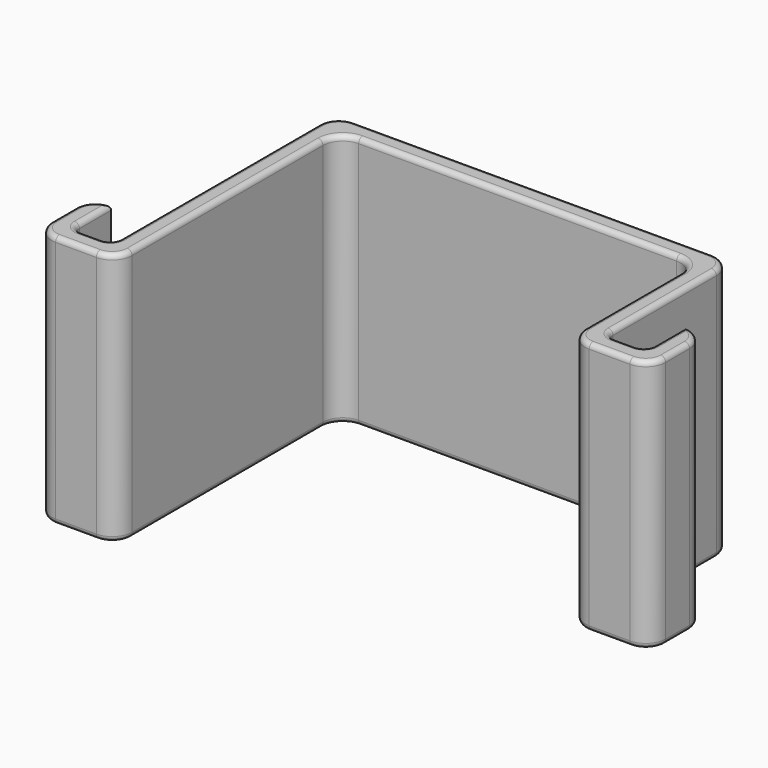
from build123d import *

# Parameters (mm, degrees)
F0_W         = 36
F0_H         = 2
F0_W_2       = 2
F0_W_3       = 4.1
F1_DEPTH     = 25.5
F2_R         = 1.99999
F3_R         = 1
F4_T1_DEPTH  = 36.00002
F4_T3_DEPTH  = 32.00002
F4_T5_DEPTH  = 25.00001
F4_T7_DEPTH  = 2.1
F4_T9_DEPTH  = 5.25
F4_T11_DEPTH = 13.00001
F4_T13_DEPTH = 1.25001
F4_T15_DEPTH = 2.1
F4_T17_DEPTH = 3.00002
F4_T19_DEPTH = 5.25
F4_T21_DEPTH = 4.10002
F4_T23_DEPTH = 1.25001
F4_T25_DEPTH = 24.00002
F4_T27_DEPTH = 3.00002
F4_T29_DEPTH = 4.10002
F4_T31_DEPTH = 12.00002
F4_T34_ANGLE = 90
F4_T36_ANGLE = 90
F4_T38_ANGLE = 90
F4_T40_ANGLE = 90
F4_T42_ANGLE = 90
F4_T44_ANGLE = 90
F4_T46_ANGLE = 90
F4_T48_ANGLE = 90
F4_T50_ANGLE = 90
F4_T52_ANGLE = 90
F4_T54_ANGLE = 90
F4_T56_ANGLE = 90
F4_T58_ANGLE = 90
F4_T60_ANGLE = 90
F4_T62_ANGLE = 90
F4_T64_ANGLE = 90
F4_T66_ANGLE = 90
F4_T68_ANGLE = 90
F4_T70_ANGLE = 90
F4_T72_ANGLE = 90
F4_T74_ANGLE = 90
F4_T76_ANGLE = 90
F4_T78_ANGLE = 90
F4_T80_ANGLE = 90
F4_T82_ANGLE = 90
F4_T84_ANGLE = 90
F4_T86_ANGLE = 90
F4_T88_ANGLE = 90


# Not quite as in the source:
# - a fillet or chamfer that OpenCascade refuses, or shapes differently, is made with other operations: its cross-section is extruded or revolved along the edge and cut away or added
# - a fillet or chamfer is up to 0.001 mm smaller than in the source, because OpenCascade refuses the exact size


with BuildPart() as f1:
    # F0 (on Top) → F1 (new body)
    with BuildSketch(Plane.XY):
        Polygon((0, -2), (0, 0), (-2, 0), (-2, -28), (0, -28), align=None)
        with Locations((18, -1)):
            Rectangle(F0_W, F0_H)
        Polygon((38, 0), (36, 0), (36, -2), (36, -16), (38, -16), align=None)
        with Locations((37, -17)):
            Rectangle(F0_W_2, F0_H)
        with Locations((40.05, -17)):
            Rectangle(F0_W_3, F0_H)
        Polygon((42.1, -11), (42.1, -16), (42.1, -18), (44.1, -18), (44.1, -11), align=None)
        Polygon((0, -30), (0, -28), (-2, -28), (-6.1, -28), (-6.1, -30), align=None)
        Polygon((-6.1, -30), (-6.1, -28), (-6.1, -23), (-8.1, -23), (-8.1, -30), align=None)
    extrude(amount=F1_DEPTH)

    # F2 (radius 2 in the source; OpenCascade refuses exactly that, so slightly less here)
    f2_edges = [f1.edges().sort_by_distance(p)[0] for p in [
        (0, -30, 12.75),
        (36, -18, 12.75),
        (-8.1, -30, 12.75),
        (44.1, -18, 12.75),
        (0, -2, 12.75),
        (36, -2, 12.75),
        (-2, 0, 12.75),
        (38, 0, 12.75),
        (44.1, -11, 12.75),
        (-8.1, -23, 12.75),
    ]]
    fillet(f2_edges, radius=F2_R)

    # F3
    f3_edges = [f1.edges().sort_by_distance(p)[0] for p in [
        (-2, -28, 12.75),
        (-6.1, -28, 12.75),
        (42.1, -16, 12.75),
        (38, -16, 12.75),
    ]]
    fillet(f3_edges, radius=F3_R)

    # F4: fillet of radius 0.5 on 58 edges, made by hand

    # F4_s2 → F4_t1 (cut)
    with BuildSketch(Plane.YZ.offset(-1e-05)):
        with BuildLine():
            ThreePointArc((-0.5, 25.5), (-0.1464466094, 25.3535533906), (0, 25))
            Line((0, 25), (0, 25.5))
            Line((0, 25.5), (-0.5, 25.5))
        make_face()
        with BuildLine():
            ThreePointArc((-0.5, 0), (-0.1464466094, 0.1464466094), (0, 0.5))
            Line((0, 0.5), (0, 0))
            Line((0, 0), (-0.5, 0))
        make_face()
    extrude(amount=F4_T1_DEPTH, mode=Mode.SUBTRACT)

    # F4_s4 → F4_t3 (cut)
    with BuildSketch(Plane.YZ.offset(1.99999)):
        with BuildLine():
            ThreePointArc((-1.5, 0), (-1.8535533906, 0.1464466094), (-2, 0.5))
            Line((-2, 0.5), (-2, 0))
            Line((-2, 0), (-1.5, 0))
        make_face()
        with BuildLine():
            ThreePointArc((-1.5, 25.5), (-1.8535533906, 25.3535533906), (-2, 25))
            Line((-2, 25), (-2, 25.5))
            Line((-2, 25.5), (-1.5, 25.5))
        make_face()
    extrude(amount=F4_T3_DEPTH, mode=Mode.SUBTRACT)

    # F4_s6 → F4_t5 (cut)
    with BuildSketch(Plane.XZ.offset(1.99999)):
        with BuildLine():
            ThreePointArc((-2, 25), (-1.8535533906, 25.3535533906), (-1.5, 25.5))
            Line((-1.5, 25.5), (-2, 25.5))
            Line((-2, 25.5), (-2, 25))
        make_face()
        with BuildLine():
            ThreePointArc((-2, 0.5), (-1.8535533906, 0.1464466094), (-1.5, 0))
            Line((-1.5, 0), (-2, 0))
            Line((-2, 0), (-2, 0.5))
        make_face()
    extrude(amount=F4_T5_DEPTH, mode=Mode.SUBTRACT)

    # F4_s8 → F4_t7 (cut)
    with BuildSketch(Plane.YZ.offset(-5.1)):
        with BuildLine():
            ThreePointArc((-28.5, 25.5), (-28.1464466094, 25.3535533906), (-28, 25))
            Line((-28, 25), (-28, 25.5))
            Line((-28, 25.5), (-28.5, 25.5))
        make_face()
        with BuildLine():
            ThreePointArc((-28.5, 0), (-28.1464466094, 0.1464466094), (-28, 0.5))
            Line((-28, 0.5), (-28, 0))
            Line((-28, 0), (-28.5, 0))
        make_face()
    extrude(amount=F4_T7_DEPTH, mode=Mode.SUBTRACT)

    # F4_s10 → F4_t9 (cut)
    with BuildSketch(Plane.XZ.offset(21.75)):
        with BuildLine():
            ThreePointArc((-6.6, 25.5), (-6.2464466094, 25.3535533906), (-6.1, 25))
            Line((-6.1, 25), (-6.1, 25.5))
            Line((-6.1, 25.5), (-6.6, 25.5))
        make_face()
        with BuildLine():
            ThreePointArc((-6.6, 0), (-6.2464466094, 0.1464466094), (-6.1, 0.5))
            Line((-6.1, 0.5), (-6.1, 0))
            Line((-6.1, 0), (-6.6, 0))
        make_face()
    extrude(amount=F4_T9_DEPTH, mode=Mode.SUBTRACT)

    # F4_s12 → F4_t11 (cut)
    with BuildSketch(Plane.XZ.offset(1.99999)):
        with BuildLine():
            ThreePointArc((37.5, 25.5), (37.8535533906, 25.3535533906), (38, 25))
            Line((38, 25), (38, 25.5))
            Line((38, 25.5), (37.5, 25.5))
        make_face()
        with BuildLine():
            ThreePointArc((37.5, 0), (37.8535533906, 0.1464466094), (38, 0.5))
            Line((38, 0.5), (38, 0))
            Line((38, 0), (37.5, 0))
        make_face()
    extrude(amount=F4_T11_DEPTH, mode=Mode.SUBTRACT)

    # F4_s14 → F4_t13 (cut)
    with BuildSketch(Plane.YZ.offset(-6.10001)):
        with BuildLine():
            ThreePointArc((-23.5, 25.5), (-23.1464466094, 25.3535533906), (-23, 25))
            Line((-23, 25), (-23, 25.5))
            Line((-23, 25.5), (-23.5, 25.5))
        make_face()
        with BuildLine():
            ThreePointArc((-23.5, 0), (-23.1464466094, 0.1464466094), (-23, 0.5))
            Line((-23, 0.5), (-23, 0))
            Line((-23, 0), (-23.5, 0))
        make_face()
    extrude(amount=F4_T13_DEPTH, mode=Mode.SUBTRACT)

    # F4_s16 → F4_t15 (cut)
    with BuildSketch(Plane.YZ.offset(39)):
        with BuildLine():
            ThreePointArc((-16.5, 25.5), (-16.1464466094, 25.3535533906), (-16, 25))
            Line((-16, 25), (-16, 25.5))
            Line((-16, 25.5), (-16.5, 25.5))
        make_face()
        with BuildLine():
            ThreePointArc((-16.5, 0), (-16.1464466094, 0.1464466094), (-16, 0.5))
            Line((-16, 0.5), (-16, 0))
            Line((-16, 0), (-16.5, 0))
        make_face()
    extrude(amount=F4_T15_DEPTH, mode=Mode.SUBTRACT)

    # F4_s18 → F4_t17 (cut)
    with BuildSketch(Plane.XZ.offset(24.99999)):
        with BuildLine():
            ThreePointArc((-7.6, 25.5), (-7.9535533906, 25.3535533906), (-8.1, 25))
            Line((-8.1, 25), (-8.1, 25.5))
            Line((-8.1, 25.5), (-7.6, 25.5))
        make_face()
        with BuildLine():
            ThreePointArc((-7.6, 0), (-7.9535533906, 0.1464466094), (-8.1, 0.5))
            Line((-8.1, 0.5), (-8.1, 0))
            Line((-8.1, 0), (-7.6, 0))
        make_face()
    extrude(amount=F4_T17_DEPTH, mode=Mode.SUBTRACT)

    # F4_s20 → F4_t19 (cut)
    with BuildSketch(Plane.XZ.offset(9.75)):
        with BuildLine():
            ThreePointArc((42.6, 25.5), (42.2464466094, 25.3535533906), (42.1, 25))
            Line((42.1, 25), (42.1, 25.5))
            Line((42.1, 25.5), (42.6, 25.5))
        make_face()
        with BuildLine():
            ThreePointArc((42.6, 0), (42.2464466094, 0.1464466094), (42.1, 0.5))
            Line((42.1, 0.5), (42.1, 0))
            Line((42.1, 0), (42.6, 0))
        make_face()
    extrude(amount=F4_T19_DEPTH, mode=Mode.SUBTRACT)

    # F4_s22 → F4_t21 (cut)
    with BuildSketch(Plane.YZ.offset(-6.10001)):
        with BuildLine():
            ThreePointArc((-29.5, 25.5), (-29.8535533906, 25.3535533906), (-30, 25))
            Line((-30, 25), (-30, 25.5))
            Line((-30, 25.5), (-29.5, 25.5))
        make_face()
        with BuildLine():
            ThreePointArc((-29.5, 0), (-29.8535533906, 0.1464466094), (-30, 0.5))
            Line((-30, 0.5), (-30, 0))
            Line((-30, 0), (-29.5, 0))
        make_face()
    extrude(amount=F4_T21_DEPTH, mode=Mode.SUBTRACT)

    # F4_s24 → F4_t23 (cut)
    with BuildSketch(Plane.YZ.offset(40.85)):
        with BuildLine():
            ThreePointArc((-11.5, 25.5), (-11.1464466094, 25.3535533906), (-11, 25))
            Line((-11, 25), (-11, 25.5))
            Line((-11, 25.5), (-11.5, 25.5))
        make_face()
        with BuildLine():
            ThreePointArc((-11.5, 0), (-11.1464466094, 0.1464466094), (-11, 0.5))
            Line((-11, 0.5), (-11, 0))
            Line((-11, 0), (-11.5, 0))
        make_face()
    extrude(amount=F4_T23_DEPTH, mode=Mode.SUBTRACT)

    # F4_s26 → F4_t25 (cut)
    with BuildSketch(Plane.XZ.offset(3.99999)):
        with BuildLine():
            ThreePointArc((-0.5, 25.5), (-0.1464466094, 25.3535533906), (0, 25))
            Line((0, 25), (0, 25.5))
            Line((0, 25.5), (-0.5, 25.5))
        make_face()
        with BuildLine():
            ThreePointArc((-0.5, 0), (-0.1464466094, 0.1464466094), (0, 0.5))
            Line((0, 0.5), (0, 0))
            Line((0, 0), (-0.5, 0))
        make_face()
    extrude(amount=F4_T25_DEPTH, mode=Mode.SUBTRACT)

    # F4_s28 → F4_t27 (cut)
    with BuildSketch(Plane.XZ.offset(12.99999)):
        with BuildLine():
            ThreePointArc((43.6, 25.5), (43.9535533906, 25.3535533906), (44.1, 25))
            Line((44.1, 25), (44.1, 25.5))
            Line((44.1, 25.5), (43.6, 25.5))
        make_face()
        with BuildLine():
            ThreePointArc((43.6, 0), (43.9535533906, 0.1464466094), (44.1, 0.5))
            Line((44.1, 0.5), (44.1, 0))
            Line((44.1, 0), (43.6, 0))
        make_face()
    extrude(amount=F4_T27_DEPTH, mode=Mode.SUBTRACT)

    # F4_s30 → F4_t29 (cut)
    with BuildSketch(Plane.YZ.offset(37.99999)):
        with BuildLine():
            ThreePointArc((-17.5, 25.5), (-17.8535533906, 25.3535533906), (-18, 25))
            Line((-18, 25), (-18, 25.5))
            Line((-18, 25.5), (-17.5, 25.5))
        make_face()
        with BuildLine():
            ThreePointArc((-17.5, 0), (-17.8535533906, 0.1464466094), (-18, 0.5))
            Line((-18, 0.5), (-18, 0))
            Line((-18, 0), (-17.5, 0))
        make_face()
    extrude(amount=F4_T29_DEPTH, mode=Mode.SUBTRACT)

    # F4_s32 → F4_t31 (cut)
    with BuildSketch(Plane.XZ.offset(3.99999)):
        with BuildLine():
            ThreePointArc((36.5, 25.5), (36.1464466094, 25.3535533906), (36, 25))
            Line((36, 25), (36, 25.5))
            Line((36, 25.5), (36.5, 25.5))
        make_face()
        with BuildLine():
            ThreePointArc((36.5, 0), (36.1464466094, 0.1464466094), (36, 0.5))
            Line((36, 0.5), (36, 0))
            Line((36, 0), (36.5, 0))
        make_face()
    extrude(amount=F4_T31_DEPTH, mode=Mode.SUBTRACT)

    # F4_s33 → F4_t34 (revolve, cut)
    with BuildSketch(Plane.XZ.offset(27)):
        with BuildLine():
            ThreePointArc((-2, 25), (-1.8535533906, 25.3535533906), (-1.5, 25.5))
            Line((-1.5, 25.5), (-2, 25.5))
            Line((-2, 25.5), (-2, 25))
        make_face()
    revolve(axis=Axis((-3, -27, 25.5), (0, 0, -1)), revolution_arc=F4_T34_ANGLE, mode=Mode.SUBTRACT)

    # F4_s35 → F4_t36 (revolve, cut)
    with BuildSketch(Plane.XZ.offset(1.99999)):
        with BuildLine():
            ThreePointArc((-2, 25), (-1.8535533906, 25.3535533906), (-1.5, 25.5))
            Line((-1.5, 25.5), (-2, 25.5))
            Line((-2, 25.5), (-2, 25))
        make_face()
    revolve(axis=Axis((-1e-05, -1.99999, 25.5), (0, 0, -1)), revolution_arc=F4_T36_ANGLE, mode=Mode.SUBTRACT)

    # F4_s37 → F4_t38 (revolve, cut)
    with BuildSketch(Plane.YZ.offset(-5.1)):
        with BuildLine():
            ThreePointArc((-28.5, 25.5), (-28.1464466094, 25.3535533906), (-28, 25))
            Line((-28, 25), (-28, 25.5))
            Line((-28, 25.5), (-28.5, 25.5))
        make_face()
    revolve(axis=Axis((-5.1, -27, 25.5), (0, 0, -1)), revolution_arc=F4_T38_ANGLE, mode=Mode.SUBTRACT)

    # F4_s39 → F4_t40 (revolve, cut)
    with BuildSketch(Plane.XZ.offset(1.99999)):
        with BuildLine():
            ThreePointArc((37.5, 25.5), (37.8535533906, 25.3535533906), (38, 25))
            Line((38, 25), (38, 25.5))
            Line((38, 25.5), (37.5, 25.5))
        make_face()
    revolve(axis=Axis((36.00001, -1.99999, 25.5), (0, 0, 1)), revolution_arc=F4_T40_ANGLE, mode=Mode.SUBTRACT)

    # F4_s41 → F4_t42 (revolve, cut)
    with BuildSketch(Plane.XZ.offset(15)):
        with BuildLine():
            ThreePointArc((37.5, 25.5), (37.8535533906, 25.3535533906), (38, 25))
            Line((38, 25), (38, 25.5))
            Line((38, 25.5), (37.5, 25.5))
        make_face()
    revolve(axis=Axis((39, -15, 25.5), (0, 0, 1)), revolution_arc=F4_T42_ANGLE, mode=Mode.SUBTRACT)

    # F4_s43 → F4_t44 (revolve, cut)
    with BuildSketch(Plane.YZ.offset(-6.10001)):
        with BuildLine():
            ThreePointArc((-23.5, 25.5), (-23.1464466094, 25.3535533906), (-23, 25))
            Line((-23, 25), (-23, 25.5))
            Line((-23, 25.5), (-23.5, 25.5))
        make_face()
    revolve(axis=Axis((-6.10001, -24.99999, 25.5), (0, 0, 1)), revolution_arc=F4_T44_ANGLE, mode=Mode.SUBTRACT)

    # F4_s45 → F4_t46 (revolve, cut)
    with BuildSketch(Plane.YZ.offset(41.1)):
        with BuildLine():
            ThreePointArc((-16.5, 25.5), (-16.1464466094, 25.3535533906), (-16, 25))
            Line((-16, 25), (-16, 25.5))
            Line((-16, 25.5), (-16.5, 25.5))
        make_face()
    revolve(axis=Axis((41.1, -15, 25.5), (0, 0, 1)), revolution_arc=F4_T46_ANGLE, mode=Mode.SUBTRACT)

    # F4_s47 → F4_t48 (revolve, cut)
    with BuildSketch(Plane.XZ.offset(28.00001)):
        with BuildLine():
            ThreePointArc((-7.6, 25.5), (-7.9535533906, 25.3535533906), (-8.1, 25))
            Line((-8.1, 25), (-8.1, 25.5))
            Line((-8.1, 25.5), (-7.6, 25.5))
        make_face()
    revolve(axis=Axis((-6.10001, -28.00001, 25.5), (0, 0, 1)), revolution_arc=F4_T48_ANGLE, mode=Mode.SUBTRACT)

    # F4_s49 → F4_t50 (revolve, cut)
    with BuildSketch(Plane.YZ.offset(-1.99999)):
        with BuildLine():
            ThreePointArc((-29.5, 25.5), (-29.8535533906, 25.3535533906), (-30, 25))
            Line((-30, 25), (-30, 25.5))
            Line((-30, 25.5), (-29.5, 25.5))
        make_face()
    revolve(axis=Axis((-1.99999, -28.00001, 25.5), (0, 0, 1)), revolution_arc=F4_T50_ANGLE, mode=Mode.SUBTRACT)

    # F4_s51 → F4_t52 (revolve, cut)
    with BuildSketch(Plane.XZ.offset(12.99999)):
        with BuildLine():
            ThreePointArc((43.6, 25.5), (43.9535533906, 25.3535533906), (44.1, 25))
            Line((44.1, 25), (44.1, 25.5))
            Line((44.1, 25.5), (43.6, 25.5))
        make_face()
    revolve(axis=Axis((42.10001, -12.99999, 25.5), (0, 0, 1)), revolution_arc=F4_T52_ANGLE, mode=Mode.SUBTRACT)

    # F4_s53 → F4_t54 (revolve, cut)
    with BuildSketch(Plane.XZ.offset(3.99999)):
        with BuildLine():
            ThreePointArc((-0.5, 25.5), (-0.1464466094, 25.3535533906), (0, 25))
            Line((0, 25), (0, 25.5))
            Line((0, 25.5), (-0.5, 25.5))
        make_face()
    revolve(axis=Axis((1.99999, -3.99999, 25.5), (0, 0, -1)), revolution_arc=F4_T54_ANGLE, mode=Mode.SUBTRACT)

    # F4_s55 → F4_t56 (revolve, cut)
    with BuildSketch(Plane.YZ.offset(42.10001)):
        with BuildLine():
            ThreePointArc((-17.5, 25.5), (-17.8535533906, 25.3535533906), (-18, 25))
            Line((-18, 25), (-18, 25.5))
            Line((-18, 25.5), (-17.5, 25.5))
        make_face()
    revolve(axis=Axis((42.10001, -16.00001, 25.5), (0, 0, 1)), revolution_arc=F4_T56_ANGLE, mode=Mode.SUBTRACT)

    # F4_s57 → F4_t58 (revolve, cut)
    with BuildSketch(Plane.YZ.offset(34.00001)):
        with BuildLine():
            ThreePointArc((-1.5, 25.5), (-1.8535533906, 25.3535533906), (-2, 25))
            Line((-2, 25), (-2, 25.5))
            Line((-2, 25.5), (-1.5, 25.5))
        make_face()
    revolve(axis=Axis((34.00001, -3.99999, 25.5), (0, 0, -1)), revolution_arc=F4_T58_ANGLE, mode=Mode.SUBTRACT)

    # F4_s59 → F4_t60 (revolve, cut)
    with BuildSketch(Plane.XZ.offset(16.00001)):
        with BuildLine():
            ThreePointArc((36.5, 25.5), (36.1464466094, 25.3535533906), (36, 25))
            Line((36, 25), (36, 25.5))
            Line((36, 25.5), (36.5, 25.5))
        make_face()
    revolve(axis=Axis((37.99999, -16.00001, 25.5), (0, 0, 1)), revolution_arc=F4_T60_ANGLE, mode=Mode.SUBTRACT)

    # F4_s61 → F4_t62 (revolve, cut)
    with BuildSketch(Plane.XZ.offset(27)):
        with BuildLine():
            ThreePointArc((-1.5, 0), (-1.8535533906, 0.1464466094), (-2, 0.5))
            Line((-2, 0.5), (-2, 0))
            Line((-2, 0), (-1.5, 0))
        make_face()
    revolve(axis=Axis((-3, -27, 0), (0, 0, -1)), revolution_arc=F4_T62_ANGLE, mode=Mode.SUBTRACT)

    # F4_s63 → F4_t64 (revolve, cut)
    with BuildSketch(Plane.XZ.offset(1.99999)):
        with BuildLine():
            ThreePointArc((-1.5, 0), (-1.8535533906, 0.1464466094), (-2, 0.5))
            Line((-2, 0.5), (-2, 0))
            Line((-2, 0), (-1.5, 0))
        make_face()
    revolve(axis=Axis((-1e-05, -1.99999, 0), (0, 0, -1)), revolution_arc=F4_T64_ANGLE, mode=Mode.SUBTRACT)

    # F4_s65 → F4_t66 (revolve, cut)
    with BuildSketch(Plane.YZ.offset(-5.1)):
        with BuildLine():
            ThreePointArc((-28.5, 0), (-28.1464466094, 0.1464466094), (-28, 0.5))
            Line((-28, 0.5), (-28, 0))
            Line((-28, 0), (-28.5, 0))
        make_face()
    revolve(axis=Axis((-5.1, -27, 0), (0, 0, -1)), revolution_arc=F4_T66_ANGLE, mode=Mode.SUBTRACT)

    # F4_s67 → F4_t68 (revolve, cut)
    with BuildSketch(Plane.XZ.offset(1.99999)):
        with BuildLine():
            ThreePointArc((37.5, 0), (37.8535533906, 0.1464466094), (38, 0.5))
            Line((38, 0.5), (38, 0))
            Line((38, 0), (37.5, 0))
        make_face()
    revolve(axis=Axis((36.00001, -1.99999, 0), (0, 0, 1)), revolution_arc=F4_T68_ANGLE, mode=Mode.SUBTRACT)

    # F4_s69 → F4_t70 (revolve, cut)
    with BuildSketch(Plane.XZ.offset(15)):
        with BuildLine():
            ThreePointArc((37.5, 0), (37.8535533906, 0.1464466094), (38, 0.5))
            Line((38, 0.5), (38, 0))
            Line((38, 0), (37.5, 0))
        make_face()
    revolve(axis=Axis((39, -15, 0), (0, 0, 1)), revolution_arc=F4_T70_ANGLE, mode=Mode.SUBTRACT)

    # F4_s71 → F4_t72 (revolve, cut)
    with BuildSketch(Plane.YZ.offset(-6.10001)):
        with BuildLine():
            ThreePointArc((-23.5, 0), (-23.1464466094, 0.1464466094), (-23, 0.5))
            Line((-23, 0.5), (-23, 0))
            Line((-23, 0), (-23.5, 0))
        make_face()
    revolve(axis=Axis((-6.10001, -24.99999, 0), (0, 0, 1)), revolution_arc=F4_T72_ANGLE, mode=Mode.SUBTRACT)

    # F4_s73 → F4_t74 (revolve, cut)
    with BuildSketch(Plane.YZ.offset(41.1)):
        with BuildLine():
            ThreePointArc((-16.5, 0), (-16.1464466094, 0.1464466094), (-16, 0.5))
            Line((-16, 0.5), (-16, 0))
            Line((-16, 0), (-16.5, 0))
        make_face()
    revolve(axis=Axis((41.1, -15, 0), (0, 0, 1)), revolution_arc=F4_T74_ANGLE, mode=Mode.SUBTRACT)

    # F4_s75 → F4_t76 (revolve, cut)
    with BuildSketch(Plane.XZ.offset(28.00001)):
        with BuildLine():
            ThreePointArc((-7.6, 0), (-7.9535533906, 0.1464466094), (-8.1, 0.5))
            Line((-8.1, 0.5), (-8.1, 0))
            Line((-8.1, 0), (-7.6, 0))
        make_face()
    revolve(axis=Axis((-6.10001, -28.00001, 0), (0, 0, 1)), revolution_arc=F4_T76_ANGLE, mode=Mode.SUBTRACT)

    # F4_s77 → F4_t78 (revolve, cut)
    with BuildSketch(Plane.YZ.offset(-1.99999)):
        with BuildLine():
            ThreePointArc((-29.5, 0), (-29.8535533906, 0.1464466094), (-30, 0.5))
            Line((-30, 0.5), (-30, 0))
            Line((-30, 0), (-29.5, 0))
        make_face()
    revolve(axis=Axis((-1.99999, -28.00001, 0), (0, 0, 1)), revolution_arc=F4_T78_ANGLE, mode=Mode.SUBTRACT)

    # F4_s79 → F4_t80 (revolve, cut)
    with BuildSketch(Plane.XZ.offset(12.99999)):
        with BuildLine():
            ThreePointArc((43.6, 0), (43.9535533906, 0.1464466094), (44.1, 0.5))
            Line((44.1, 0.5), (44.1, 0))
            Line((44.1, 0), (43.6, 0))
        make_face()
    revolve(axis=Axis((42.10001, -12.99999, 0), (0, 0, 1)), revolution_arc=F4_T80_ANGLE, mode=Mode.SUBTRACT)

    # F4_s81 → F4_t82 (revolve, cut)
    with BuildSketch(Plane.XZ.offset(3.99999)):
        with BuildLine():
            ThreePointArc((-0.5, 0), (-0.1464466094, 0.1464466094), (0, 0.5))
            Line((0, 0.5), (0, 0))
            Line((0, 0), (-0.5, 0))
        make_face()
    revolve(axis=Axis((1.99999, -3.99999, 0), (0, 0, -1)), revolution_arc=F4_T82_ANGLE, mode=Mode.SUBTRACT)

    # F4_s83 → F4_t84 (revolve, cut)
    with BuildSketch(Plane.YZ.offset(42.10001)):
        with BuildLine():
            ThreePointArc((-17.5, 0), (-17.8535533906, 0.1464466094), (-18, 0.5))
            Line((-18, 0.5), (-18, 0))
            Line((-18, 0), (-17.5, 0))
        make_face()
    revolve(axis=Axis((42.10001, -16.00001, 0), (0, 0, 1)), revolution_arc=F4_T84_ANGLE, mode=Mode.SUBTRACT)

    # F4_s85 → F4_t86 (revolve, cut)
    with BuildSketch(Plane.YZ.offset(34.00001)):
        with BuildLine():
            ThreePointArc((-1.5, 0), (-1.8535533906, 0.1464466094), (-2, 0.5))
            Line((-2, 0.5), (-2, 0))
            Line((-2, 0), (-1.5, 0))
        make_face()
    revolve(axis=Axis((34.00001, -3.99999, 0), (0, 0, -1)), revolution_arc=F4_T86_ANGLE, mode=Mode.SUBTRACT)

    # F4_s87 → F4_t88 (revolve, cut)
    with BuildSketch(Plane.XZ.offset(16.00001)):
        with BuildLine():
            ThreePointArc((36.5, 0), (36.1464466094, 0.1464466094), (36, 0.5))
            Line((36, 0.5), (36, 0))
            Line((36, 0), (36.5, 0))
        make_face()
    revolve(axis=Axis((37.99999, -16.00001, 0), (0, 0, 1)), revolution_arc=F4_T88_ANGLE, mode=Mode.SUBTRACT)


solid = f1.part
